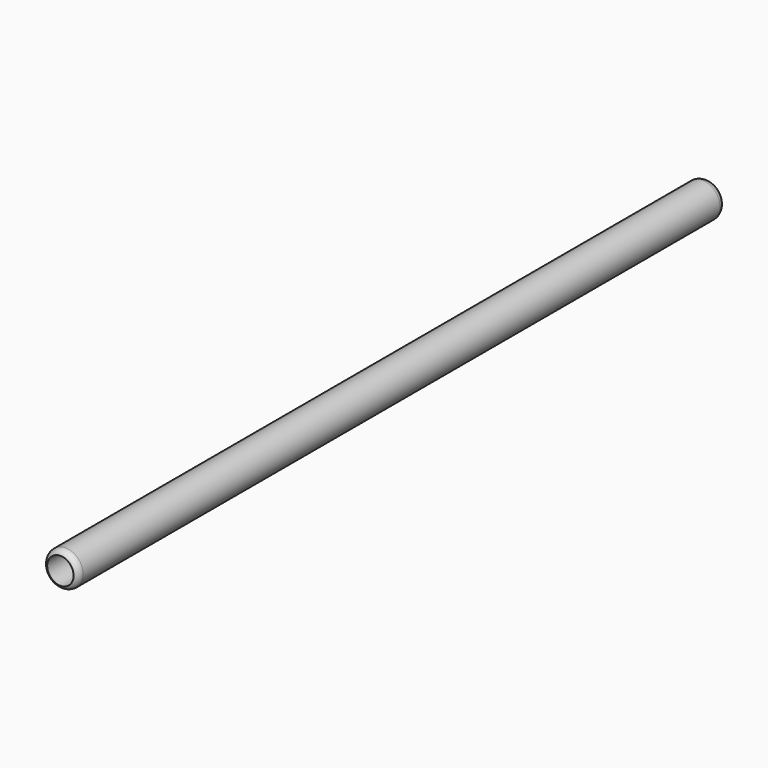
from build123d import *

# Parameters (mm, degrees)
F0_R     = 12.7
F1_DEPTH = 584.2
F2_R     = 9.525
F3_DEPTH = 584.201


# Not quite as in the source:
# - a fillet or chamfer that OpenCascade refuses, or shapes differently, is made with other operations: its cross-section is extruded or revolved along the edge and cut away or added


with BuildPart() as f1:
    # F0 (on Front) → F1 (new body)
    with BuildSketch(Plane.XZ):
        Circle(F0_R)
    extrude(amount=F1_DEPTH)

    # F2 (on face) → F3 (cut, through all)
    with BuildSketch(Plane.XZ.offset(584.2)):
        Circle(F2_R)
    extrude(amount=-F3_DEPTH, mode=Mode.SUBTRACT)

    # F4: fillet of radius 5.08 on 2 edges, made by hand

    # F4_s1 → F4_t2 (revolve, cut)
    with BuildSketch(Plane.XY):
        with BuildLine():
            ThreePointArc((12.7, -579.4907139607), (11.8321134838, -582.3305202921), (9.525, -584.2))
            Line((9.525, -584.2), (12.7, -584.2))
            Line((12.7, -584.2), (12.7, -579.4907139607))
        make_face()
    revolve(axis=Axis((0, -584.2, 0), (0, -1, 0)), mode=Mode.SUBTRACT)

    # F4_s3 → F4_t4 (revolve, cut)
    with BuildSketch(Plane.XY):
        with BuildLine():
            ThreePointArc((12.7, -4.7092860393), (11.8321134838, -1.8694797079), (9.525, 0))
            Line((9.525, 0), (12.7, 0))
            Line((12.7, 0), (12.7, -4.7092860393))
        make_face()
    revolve(axis=Axis((0, 0, 0), (0, -1, 0)), mode=Mode.SUBTRACT)


solid = f1.part
